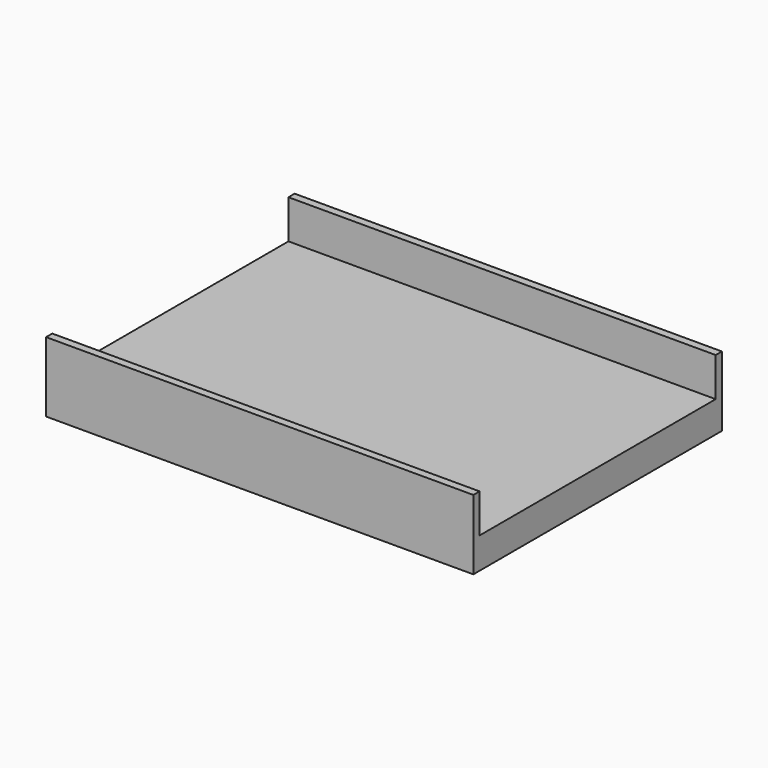
from build123d import *

# Parameters (mm, degrees)
F0_W     = 55
F0_H     = 40
F1_DEPTH = 4
F2_W     = 55
F2_H     = 1
F3_DEPTH = 5
F4_W     = 55
F4_H     = 1
F5_DEPTH = 5


# Not quite as in the source:
# - the program builds the solid bodies; features that only make, move or delete a surface that nothing else refers to are left out


with BuildPart() as f1:
    # F0 (on Top) → F1 (new body)
    with BuildSketch(Plane.XY):
        Rectangle(F0_W, F0_H)
    extrude(amount=F1_DEPTH)

    # F2 (on face) → F3 (join)
    with BuildSketch(Plane.XY.offset(4)):
        with Locations((0, -19.5)):
            Rectangle(F2_W, F2_H)
    extrude(amount=F3_DEPTH)

    # F4 (on face) → F5 (join)
    with BuildSketch(Plane.XY.offset(4)):
        with Locations((0, 19.5)):
            Rectangle(F4_W, F4_H)
    extrude(amount=F5_DEPTH)


solid = f1.part
